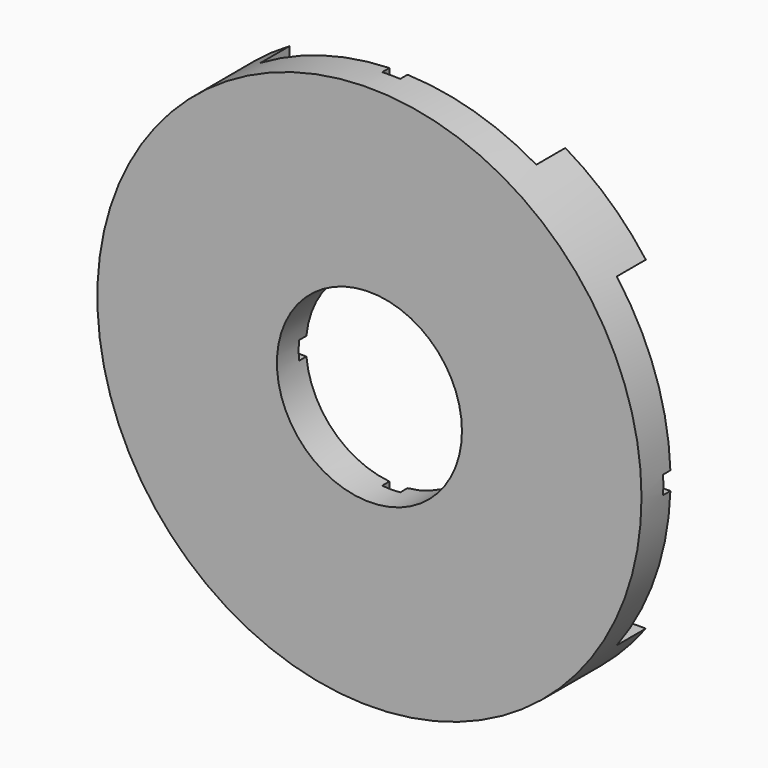
from build123d import *

# Parameters (mm, degrees)
F0_R          = 12.7
F1_DEPTH      = 17.78
F2_R          = 38.1
F3_DEPTH      = 10.16
F4_R          = 12.954
F5_DEPTH      = 17.781
F5_DEPTH_BACK = 115
F6_W          = 5.08
F6_H          = 45.466
F7_DEPTH      = 38.101
F7_DEPTH_BACK = 38.101
F8_W          = 38.608
F8_H          = 5.08
F9_DEPTH      = 38.101
F9_DEPTH_BACK = 38.101
F11_DEPTH     = 6.35


# Not quite as in the source:
# - an extrude ends at something that could not be found from the text; its depth is read off the source's solid


with BuildPart() as f1:
    # F0 (on Front) → F1 (new body)
    with BuildSketch(Plane.XZ):
        Circle(F0_R)
    extrude(amount=F1_DEPTH)

    # F2 (on Front) → F3 (join)
    with BuildSketch(Plane.XZ):
        Circle(F2_R)
    extrude(amount=F3_DEPTH)

    # F4 (on Front) → F5 (cut, two sides)
    with BuildSketch(Plane.XZ) as f5_sk:
        Circle(F4_R)
    extrude(amount=F5_DEPTH, mode=Mode.SUBTRACT)
    extrude(f5_sk.sketch, amount=-F5_DEPTH_BACK, mode=Mode.SUBTRACT)

    # F6 (on Right) → F7 (cut, two sides)
    with BuildSketch(Plane.YZ) as f7_sk:
        with Locations((-2.54, 0)):
            Rectangle(F6_W, F6_H)
    extrude(amount=F7_DEPTH, mode=Mode.SUBTRACT)
    extrude(f7_sk.sketch, amount=-F7_DEPTH_BACK, mode=Mode.SUBTRACT)

    # F8 (on Top) → F9 (cut, two sides)
    with BuildSketch(Plane.XY) as f9_sk:
        with Locations((0, -2.54)):
            Rectangle(F8_W, F8_H)
    extrude(amount=-F9_DEPTH, mode=Mode.SUBTRACT)
    extrude(f9_sk.sketch, amount=F9_DEPTH_BACK, mode=Mode.SUBTRACT)

    # F10 (on face) → F11 (cut)
    with BuildSketch(Plane(origin=(0, 0, 0), x_dir=(-1, 0, 0), z_dir=(0, 1, 0))):
        with BuildLine():
            Line((1.27, -1.27), (38.0788274504, -1.27))
            ThreePointArc((38.0788274504, -1.27), (38.1, 0), (38.0788274504, 1.27))
            Line((38.0788274504, 1.27), (1.27, 1.27))
            Line((1.27, 1.27), (1.27, 38.0788274504))
            ThreePointArc((1.27, 38.0788274504), (0, 38.1), (-1.27, 38.0788274504))
            Line((-1.27, 38.0788274504), (-1.27, 1.27))
            Line((-1.27, 1.27), (-38.0788274504, 1.27))
            ThreePointArc((-38.0788274504, 1.27), (-38.1, 0), (-38.0788274504, -1.27))
            Line((-38.0788274504, -1.27), (-1.27, -1.27))
            Line((-1.27, -1.27), (-1.27, -38.0788274504))
            ThreePointArc((-1.27, -38.0788274504), (0, -38.1), (1.27, -38.0788274504))
            Line((1.27, -38.0788274504), (1.27, -1.27))
        make_face()
    extrude(amount=-F11_DEPTH, mode=Mode.SUBTRACT)


solid = f1.part
